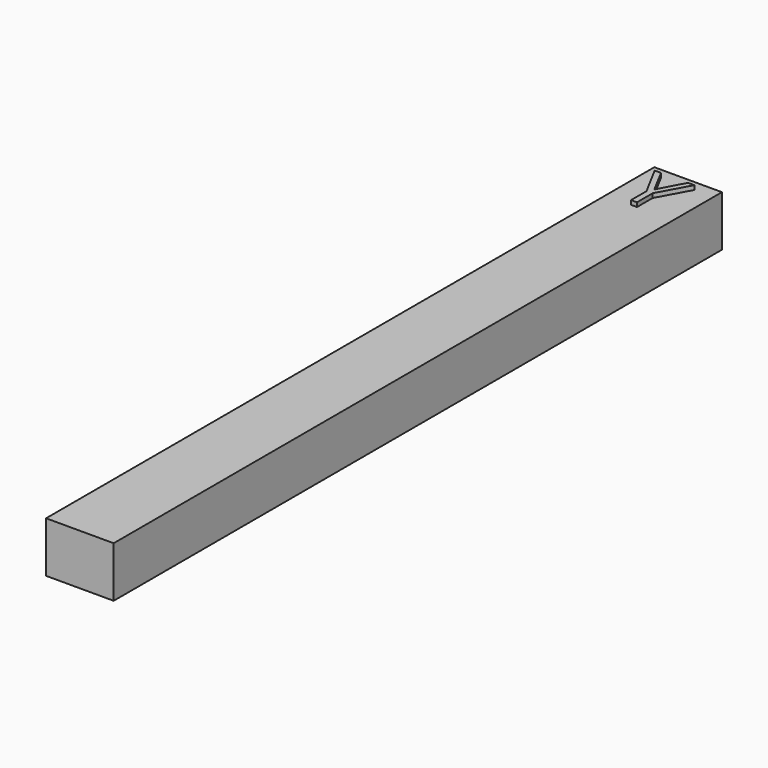
from build123d import *

# Parameters (mm, degrees)
F0_W         = 8
F0_H         = 6
F1_DEPTH     = 90
F2_TEXT_SIZE = 8.3768428239
F3_DEPTH     = 0.5


# Not quite as in the source:
# - Text() gives the source's letters only with a copy of the font that has no kerning and outlines rounded to 1/6400 em; it was checked with that copy


with BuildPart() as f1:
    # F0 (on Front) → F1 (new body)
    with BuildSketch(Plane.XZ):
        Rectangle(F0_W, F0_H)
    extrude(amount=F1_DEPTH)

    # F2 (on face) → F3 (join)
    with BuildSketch(Plane.XY.offset(3)):
        with Locations((-2.9592730571, -7.2361961938)):
            Text('Y', F2_TEXT_SIZE, font='Open Sans', text_align=(TextAlign.LEFT, TextAlign.BOTTOM))
    extrude(amount=F3_DEPTH)


solid = f1.part
